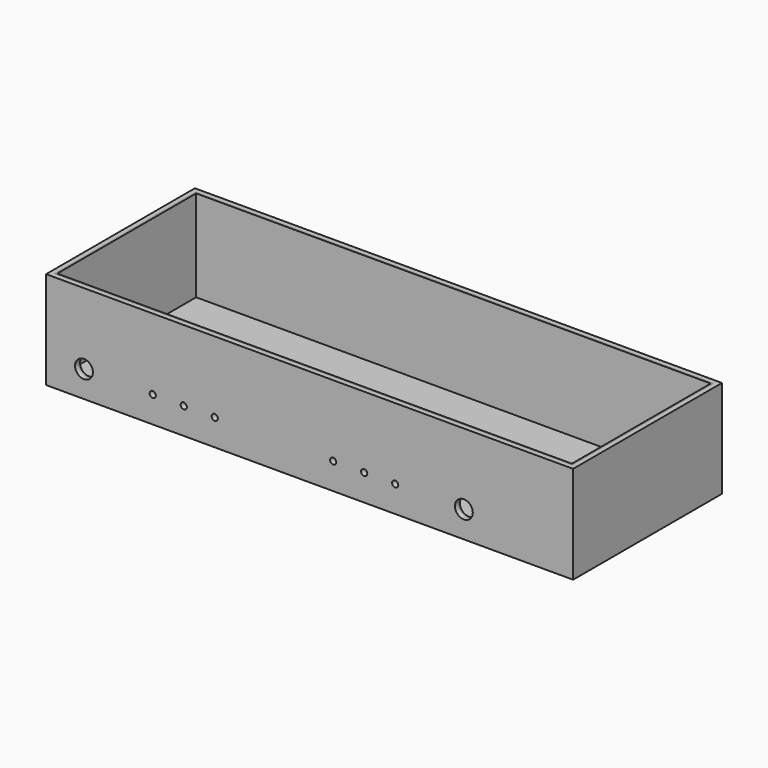
from build123d import *

# Parameters (mm, degrees)
F0_W     = 850
F0_H     = 300
F1_DEPTH = 7.5
F2_W     = 850
F2_H     = 300
F2_W_2   = 835
F2_H_2   = 285
F3_DEPTH = 150
F4_DEPTH = 2.5
F5_W     = 835
F5_H     = 285
F5_W_2   = 830
F5_H_2   = 280
F6_DEPTH = 147.5
F7_R     = 5
F7_R_2   = 14.39
F8_DEPTH = 25


with BuildPart() as f1:
    # F0 (on Top) → F1 (new body)
    with BuildSketch(Plane.XY):
        Rectangle(F0_W, F0_H)
    extrude(amount=F1_DEPTH)

    # F2 (on face) → F3 (join)
    with BuildSketch(Plane.XY.offset(7.5)):
        Rectangle(F2_W, F2_H)
        Rectangle(F2_W_2, F2_H_2, mode=Mode.SUBTRACT)
    extrude(amount=F3_DEPTH)


with BuildPart() as f4:
    # F4 (new): a face of the model
    f4_faces = [f1.part.faces().sort_by_distance(p)[0] for p in [
        (0, 0, 7.5),
    ]]
    extrude(f4_faces, amount=F4_DEPTH)

    # F5 (on face) → F6 (join)
    with BuildSketch(Plane.XY.offset(10)):
        Rectangle(F5_W, F5_H)
        Rectangle(F5_W_2, F5_H_2, mode=Mode.SUBTRACT)
    extrude(amount=F6_DEPTH)


with BuildPart() as f8_tool:
    # F7 (on face) → F8 (new body)
    with BuildSketch(Plane.XZ.offset(150)):
        with Locations((-153, 42.655)):
            Circle(F7_R)
        with Locations((38, 42.655)):
            Circle(F7_R)
        with Locations((88, 42.655)):
            Circle(F7_R)
        with Locations((138, 42.655)):
            Circle(F7_R)
        with Locations((-203, 42.655)):
            Circle(F7_R)
        with Locations((-253, 42.655)):
            Circle(F7_R)
        with Locations((248.784, 42.655)):
            Circle(F7_R_2)
        with Locations((-363.843, 42.655)):
            Circle(F7_R_2)
    extrude(amount=-F8_DEPTH)


with BuildPart() as f1_1:
    add(f1.part)

    # F8: cut by f8_tool
    add(f8_tool.part, mode=Mode.SUBTRACT)


with BuildPart() as f4_1:
    add(f4.part)

    # F8: cut by f8_tool
    add(f8_tool.part, mode=Mode.SUBTRACT)


solid = Compound([f1_1.part, f4_1.part])
